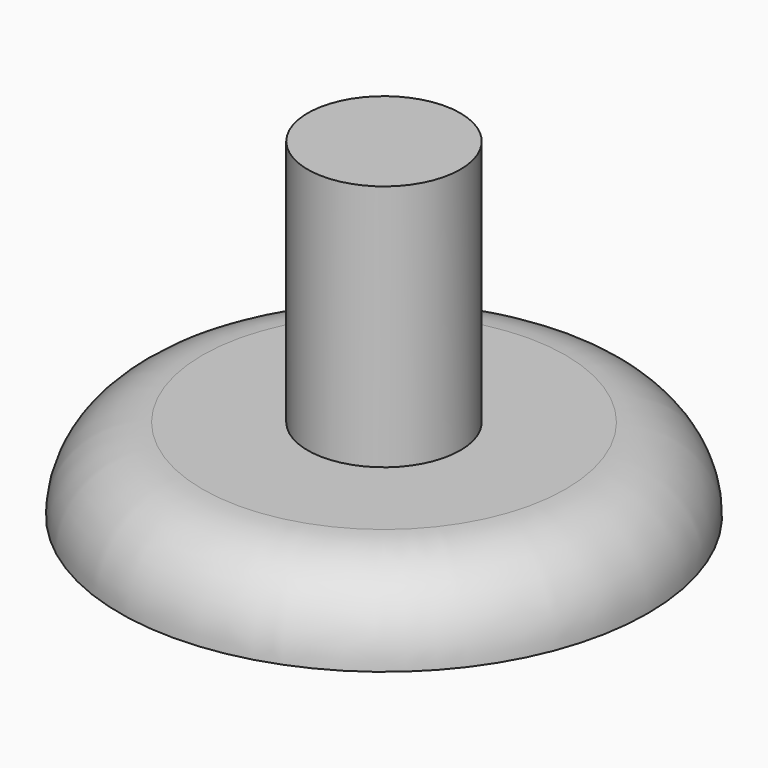
from build123d import *

# Parameters (mm, degrees)
F0_R     = 40.6727472004
F0_R_2   = 11.7636370253
F1_DEPTH = 12.7
F2_R     = 12.69999
F3_DEPTH = 50.8


# Not quite as in the source:
# - a fillet or chamfer is up to 0.001 mm smaller than in the source, because OpenCascade refuses the exact size
# - the program builds the solid bodies; features that only make, move or delete a surface that nothing else refers to are left out


with BuildPart() as f1:
    # F0 (on Top) → F1 (new body)
    with BuildSketch(Plane.XY):
        Circle(F0_R)
        Circle(F0_R_2, mode=Mode.SUBTRACT)
    extrude(amount=F1_DEPTH)

    # F2 (radius 12.7 in the source; OpenCascade refuses exactly that, so slightly less here)
    f2_edges = [f1.edges().sort_by_distance(p)[0] for p in [
        (-40.672747, 0, 12.7),
    ]]
    fillet(f2_edges, radius=F2_R)

    # F0 (on Top) → F3 (join)
    with BuildSketch(Plane.XY):
        Circle(F0_R_2)
    extrude(amount=F3_DEPTH)


solid = f1.part
